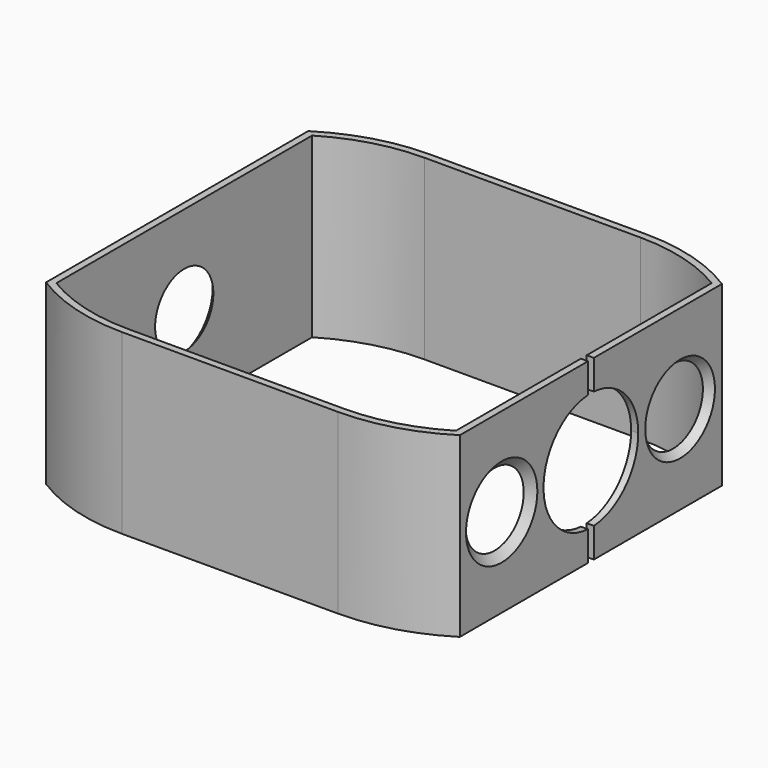
from build123d import *

# Parameters (mm, degrees)
F1_DEPTH = 9.525
F2_R     = 3.90906
F3_DEPTH = 25.4
F4_DEPTH = 25.4
F5_R     = 3.90525
F6_DEPTH = 25.4


# Not quite as in the source:
# - a fillet or chamfer that OpenCascade refuses, or shapes differently, is made with other operations: its cross-section is extruded or revolved along the edge and cut away or added


with BuildPart() as f1:
    # F0 (on Top) → F1 (new body, symmetric)
    with BuildSketch(Plane.XY):
        with BuildLine():
            Line((0, 20.6466445854), (-11.58875, 20.6466445854))
            ThreePointArc((-11.58875, 20.6466445854), (-17.1096965819, 19.861848606), (-22.19325, 17.5696355848))
            Line((-22.19325, 17.5696355848), (-22.19325, -17.5696355848))
            ThreePointArc((-22.19325, -17.5696355848), (-17.1096965819, -19.861848606), (-11.58875, -20.6466445854))
            Line((-11.58875, -20.6466445854), (0, -20.6466445854))
            Line((0, -20.6466445854), (11.58875, -20.6466445854))
            ThreePointArc((11.58875, -20.6466445854), (17.1096965819, -19.861848606), (22.19325, -17.5696355848))
            Line((22.19325, -17.5696355848), (22.19325, 17.5696355848))
            ThreePointArc((22.19325, 17.5696355848), (17.1096965819, 19.861848606), (11.58875, 20.6466445854))
            Line((11.58875, 20.6466445854), (0, 20.6466445854))
        make_face()
        with BuildLine():
            ThreePointArc((11.58875, 19.8846445854), (16.6970877606, 19.1869573913), (21.43125, 17.145))
            Line((21.43125, 17.145), (21.43125, -17.145))
            ThreePointArc((21.43125, -17.145), (16.6970877606, -19.1869573913), (11.58875, -19.8846445854))
            Line((11.58875, -19.8846445854), (0, -19.8846445854))
            Line((0, -19.8846445854), (-11.58875, -19.8846445854))
            ThreePointArc((-11.58875, -19.8846445854), (-16.6970877606, -19.1869573913), (-21.43125, -17.145))
            Line((-21.43125, -17.145), (-21.43125, 17.145))
            ThreePointArc((-21.43125, 17.145), (-16.6970877606, 19.1869573913), (-11.58875, 19.8846445854))
            Line((-11.58875, 19.8846445854), (0, 19.8846445854))
            Line((0, 19.8846445854), (11.58875, 19.8846445854))
        make_face(mode=Mode.SUBTRACT)
    extrude(amount=F1_DEPTH, both=True)

    # F2 (on face) → F3 (cut)
    with BuildSketch(Plane.YZ.offset(22.19325)):
        with BuildLine():
            ThreePointArc((0.396875, -6.3375855209), (4.6283180665, -4.3475478002), (6.35, 0))
            ThreePointArc((6.35, 0), (4.6283180665, 4.3475478002), (0.396875, 6.3375855209))
            Line((0.396875, 6.3375855209), (0.396875, -6.3375855209))
        make_face()
        with BuildLine():
            Line((0.396875, -6.3375855209), (0.396875, 6.3375855209))
            ThreePointArc((0.396875, 6.3375855209), (0, 6.35), (-0.396875, 6.3375855209))
            Line((-0.396875, 6.3375855209), (-0.396875, -6.3375855209))
            ThreePointArc((-0.396875, -6.3375855209), (0, -6.35), (0.396875, -6.3375855209))
        make_face()
        with BuildLine():
            ThreePointArc((-0.396875, 6.3375855209), (0, 6.35), (0.396875, 6.3375855209))
            Line((0.396875, 6.3375855209), (0.396875, 16.235569492))
            Line((0.396875, 16.235569492), (-0.396875, 16.235569492))
            Line((-0.396875, 16.235569492), (-0.396875, 6.3375855209))
        make_face()
        with BuildLine():
            Line((0.396875, -16.235569492), (0.396875, -6.3375855209))
            ThreePointArc((0.396875, -6.3375855209), (0, -6.35), (-0.396875, -6.3375855209))
            Line((-0.396875, -6.3375855209), (-0.396875, -16.235569492))
            Line((-0.396875, -16.235569492), (0.396875, -16.235569492))
        make_face()
        with BuildLine():
            Line((-0.396875, -6.3375855209), (-0.396875, 6.3375855209))
            ThreePointArc((-0.396875, 6.3375855209), (-6.35, 0), (-0.396875, -6.3375855209))
        make_face()
        with Locations((-11.9634, 0)):
            Circle(F2_R)
        with Locations((11.9634, 0)):
            Circle(F2_R)
    extrude(amount=-F3_DEPTH, mode=Mode.SUBTRACT)

    # F2 (on face) → F4 (cut)
    with BuildSketch(Plane.YZ.offset(22.19325)):
        with BuildLine():
            ThreePointArc((0.396875, -6.3375855209), (4.6283180665, -4.3475478002), (6.35, 0))
            ThreePointArc((6.35, 0), (4.6283180665, 4.3475478002), (0.396875, 6.3375855209))
            Line((0.396875, 6.3375855209), (0.396875, -6.3375855209))
        make_face()
        with BuildLine():
            Line((0.396875, -6.3375855209), (0.396875, 6.3375855209))
            ThreePointArc((0.396875, 6.3375855209), (0, 6.35), (-0.396875, 6.3375855209))
            Line((-0.396875, 6.3375855209), (-0.396875, -6.3375855209))
            ThreePointArc((-0.396875, -6.3375855209), (0, -6.35), (0.396875, -6.3375855209))
        make_face()
        with BuildLine():
            ThreePointArc((-0.396875, 6.3375855209), (0, 6.35), (0.396875, 6.3375855209))
            Line((0.396875, 6.3375855209), (0.396875, 16.235569492))
            Line((0.396875, 16.235569492), (-0.396875, 16.235569492))
            Line((-0.396875, 16.235569492), (-0.396875, 6.3375855209))
        make_face()
        with BuildLine():
            Line((0.396875, -16.235569492), (0.396875, -6.3375855209))
            ThreePointArc((0.396875, -6.3375855209), (0, -6.35), (-0.396875, -6.3375855209))
            Line((-0.396875, -6.3375855209), (-0.396875, -16.235569492))
            Line((-0.396875, -16.235569492), (0.396875, -16.235569492))
        make_face()
        with BuildLine():
            Line((-0.396875, -6.3375855209), (-0.396875, 6.3375855209))
            ThreePointArc((-0.396875, 6.3375855209), (-6.35, 0), (-0.396875, -6.3375855209))
        make_face()
        with Locations((-11.9634, 0)):
            Circle(F2_R)
        with Locations((11.9634, 0)):
            Circle(F2_R)
    extrude(amount=-F4_DEPTH, mode=Mode.SUBTRACT)

    # F5 (on face) → F6 (cut)
    with BuildSketch(Plane(origin=(-22.19325, 0, 0), x_dir=(0, -1, 0), z_dir=(-1, 0, 0))):
        Circle(F5_R)
    extrude(amount=-F6_DEPTH, mode=Mode.SUBTRACT)

    # F7: chamfer of 0.762 x 0.8765807263 on 3 edges, made by hand

    # F7_s1 → F7_t2 (revolve, cut)
    with BuildSketch(Plane.XY):
        Polygon((22.19325, -7.1777592737), (21.43125, -8.05434), (22.19325, -8.05434), align=None)
    revolve(axis=Axis((22.19325, -11.9634, 0), (1, 0, 0)), mode=Mode.SUBTRACT)

    # F7_s3 → F7_t4 (revolve, cut)
    with BuildSketch(Plane.XY):
        Polygon((22.19325, 16.63446), (21.3166692737, 15.87246), (22.19325, 15.87246), align=None)
    revolve(axis=Axis((22.19325, 11.9634, 0), (1, 0, 0)), mode=Mode.SUBTRACT)

    # F7_s5 → F7_t6 (revolve, cut)
    with BuildSketch(Plane.XY):
        Polygon((-22.19325, -4.7818307263), (-21.43125, -3.90525), (-22.19325, -3.90525), align=None)
    revolve(axis=Axis((-22.19325, 0, 0), (-1, 0, 0)), mode=Mode.SUBTRACT)


solid = f1.part
